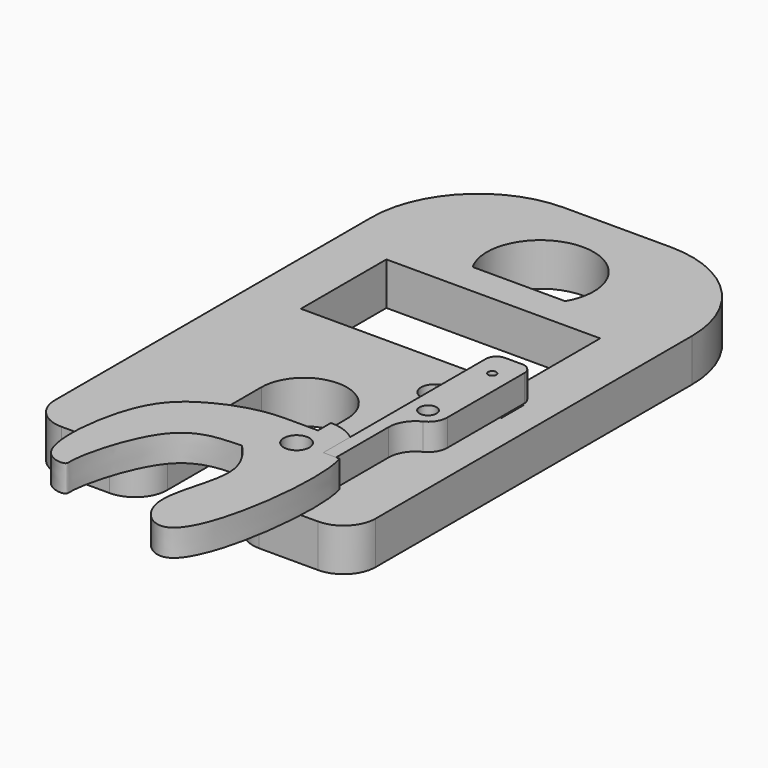
from build123d import *

# Parameters (mm, degrees)
F0_R      = 1.524
F1_DEPTH  = 3.175
F2_R      = 0.635
F3_DEPTH  = 5.08
F4_R      = 1.016
F4_R_2    = 0.4765946888
F5_DEPTH  = 3.175
F6_D      = 1.016
F8_DEPTH  = 25.4
F9_W      = 25.4
F9_H      = 12.7
F10_DEPTH = 25.4


with BuildPart() as f1:
    # F0 (on Top) → F1 (new body)
    with BuildSketch(Plane.XY):
        with BuildLine():
            add(Edge.make_bspline(
                [(4.0146798487, 4.0146798487), (4.1965253446, 3.8388911287), (8.6034145204, -0.4632855785), (2.7081005667, -9.8256704348), (11.7725199973, -17.5553609081), (14.1365779009, 3.6148799922), (12.7186926547, 7.62)],
                knots=[0.342546698, 0.342546698, 0.342546698, 0.342546698, 0.4592804701, 0.6325061967, 0.7529179928, 1, 1, 1, 1], degree=3))
            Line((12.7186926547, 7.62), (10.795, 7.62))
            Line((10.795, 7.62), (10.795, 11.6094914196))
            ThreePointArc((10.795, 11.6094914196), (9.3015879683, 12.4334113363), (7.62, 12.7186926547))
            Line((7.62, 12.7186926547), (7.62, 10.795))
            Line((7.62, 10.795), (3.6305085804, 10.795))
            add(Edge.make_bspline(
                [(-9.8462747246, -2.5595309993), (-9.7056248656, -0.6525965961), (-8.5851336869, 4.887523046), (-4.9223199156, 8.8010582074), (0.6214204647, 10.795), (3.6305085804, 10.795)],
                knots=[0.5944478908, 0.5944478908, 0.5944478908, 0.5944478908, 0.6806042793, 0.8326685389, 1, 1, 1, 1], degree=3))
            add(Edge.make_bspline(
                [(-9.8462747246, -2.5595309993), (-8.3692950914, 1.0159390836), (-1.2709087492, 7.2679963496), (3.9839462531, 4.0422517138), (3.9949946041, 4.0337094316), (4.0146798487, 4.0146798487)],
                knots=[0.0522687231, 0.0522687231, 0.0522687231, 0.0522687231, 0.2064144516, 0.3299099657, 0.342546698, 0.342546698, 0.342546698, 0.342546698], degree=3))
        make_face()
        with Locations((7.62, 7.62)):
            Circle(F0_R, mode=Mode.SUBTRACT)
        with BuildLine():
            add(Edge.make_bspline(
                [(4.0146798487, 4.0146798487), (1.5786877312, 3.9404286991), (-3.8406877482, 3.7898553775), (-6.77720019, -7.7849709454), (-6.196463978, -9.2958597248), (-9.5973471823, -8.9863377062), (-10.0193170502, -4.9056432962), (-9.8462747246, -2.5595309993)],
                knots=[0, 0, 0, 0, 0.1532538956, 0.3403377332, 0.3978065221, 0.4884491935, 0.5944478908, 0.5944478908, 0.5944478908, 0.5944478908], degree=3))
            add(Edge.make_bspline(
                [(-9.8462747246, -2.5595309993), (-8.3692950914, 1.0159390836), (-1.2709087492, 7.2679963496), (3.9839462531, 4.0422517138), (3.9949946041, 4.0337094316), (4.0146798487, 4.0146798487)],
                knots=[0.0522687231, 0.0522687231, 0.0522687231, 0.0522687231, 0.2064144516, 0.3299099657, 0.342546698, 0.342546698, 0.342546698, 0.342546698], degree=3))
        make_face()
    extrude(amount=F1_DEPTH)


with BuildPart() as f3:
    # F2 (on Top) → F3 (new body)
    with BuildSketch(Plane.XY):
        with BuildLine():
            Line((6.35, 64.77), (-6.35, 64.77))
            ThreePointArc((-6.35, 64.77), (-15.3302561211, 61.0502561211), (-19.05, 52.07))
            Line((-19.05, 52.07), (-19.05, 5.08))
            ThreePointArc((-19.05, 5.08), (-17.9340768363, 2.3859231637), (-15.24, 1.27))
            Line((-15.24, 1.27), (-9.525, 1.27))
            ThreePointArc((-9.525, 1.27), (-6.8309231637, 2.3859231637), (-5.715, 5.08))
            Line((-5.715, 5.08), (-5.715, 19.05))
            ThreePointArc((-5.715, 19.05), (-0.635, 24.13), (4.445, 19.05))
            Line((4.445, 19.05), (4.445, 5.08))
            ThreePointArc((4.445, 5.08), (5.5609231637, 2.3859231637), (8.255, 1.27))
            Line((8.255, 1.27), (15.24, 1.27))
            ThreePointArc((15.24, 1.27), (17.9340768363, 2.3859231637), (19.05, 5.08))
            Line((19.05, 5.08), (19.05, 52.07))
            ThreePointArc((19.05, 52.07), (15.3302561211, 61.0502561211), (6.35, 64.77))
        make_face()
        with Locations((7.62, 7.62)):
            Circle(F2_R, mode=Mode.SUBTRACT)
        with BuildLine():
            ThreePointArc((-5.499261314, 50.165), (0, 59.69), (5.499261314, 50.165))
            Line((5.499261314, 50.165), (-5.499261314, 50.165))
        make_face(mode=Mode.SUBTRACT)
    extrude(amount=-F3_DEPTH)

    # F6 (through all)
    with Locations(Plane.XY):
        with Locations((13.081, 20.32)):
            Hole(F6_D / 2)

    # F7 (on face) → F8 (cut)
    with BuildSketch(Plane.XY):
        with BuildLine():
            Line((15.5435356842, 28.1201432546), (15.5435356842, 31.4043808392))
            ThreePointArc((15.5435356842, 31.4043808392), (10.8526970709, 31.4538334208), (6.542203401, 29.6028723799))
            ThreePointArc((6.542203401, 29.6028723799), (6.1585518853, 27.3908316899), (8.3705925754, 27.0071801742))
            ThreePointArc((8.3705925754, 27.0071801742), (11.826845486, 28.4029087118), (15.5435356842, 28.1201432546))
        make_face()
    extrude(amount=-F8_DEPTH, mode=Mode.SUBTRACT)

    # F9 (on face) → F10 (cut)
    with BuildSketch(Plane.XY):
        with Locations((0, 40.005)):
            Rectangle(F9_W, F9_H)
    extrude(amount=-F10_DEPTH, mode=Mode.SUBTRACT)


with BuildPart() as f5:
    # F4 (on face) → F5 (new body)
    with BuildSketch(Plane.XY):
        with BuildLine():
            Line((10.795, 31.75), (10.795, 7.62))
            Line((10.795, 7.62), (12.319, 7.62))
            Line((12.319, 7.62), (12.319, 15.4210254134))
            ThreePointArc((12.319, 15.4210254134), (12.7981833657, 17.09828439), (14.0910930233, 18.2692664521))
            ThreePointArc((14.0910930233, 18.2692664521), (15.0219879767, 19.1123735369), (15.367, 20.32))
            Line((15.367, 20.32), (15.367, 31.75))
            ThreePointArc((15.367, 31.75), (14.9950256121, 32.6480256121), (14.097, 33.02))
            Line((14.097, 33.02), (12.065, 33.02))
            ThreePointArc((12.065, 33.02), (11.1669743879, 32.6480256121), (10.795, 31.75))
        make_face()
        with Locations((13.081, 20.32)):
            Circle(F4_R, mode=Mode.SUBTRACT)
        with Locations((13.081, 29.845)):
            Circle(F4_R_2, mode=Mode.SUBTRACT)
    extrude(amount=F5_DEPTH)


solid = Compound([f1.part, f3.part, f5.part])
